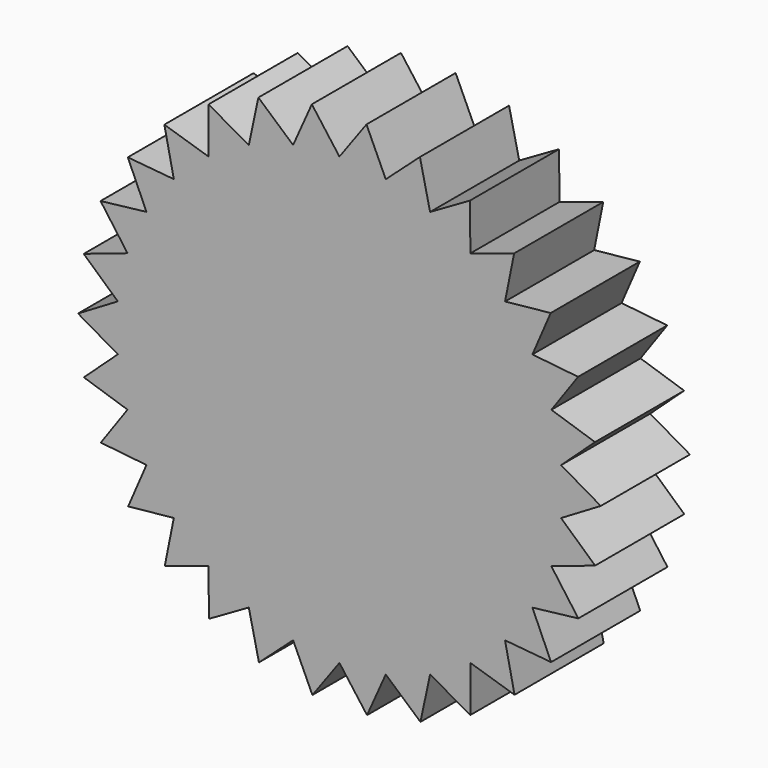
from build123d import *

# Parameters (mm, degrees)
F0_R            = 50.8
F1_DEPTH        = 12.7
F3_DEPTH        = 25.4
F3_COPIES_COUNT = 30


# Not quite as in the source:
# - a pattern or mirror of a feature is missing from the dataset's text; its kind, count and spacing are read off the source's solid


with BuildPart() as f1:
    # F0 (on Front) → F1 (new body, symmetric)
    with BuildSketch(Plane.XZ):
        Circle(F0_R)
    extrude(amount=F1_DEPTH, both=True)

    # F2 (on face) → F3 (join)
    with BuildSketch(Plane.XZ.offset(12.7)):
        with BuildLine():
            ThreePointArc((0, 50.8), (5.310045934, 50.5217122847), (10.5619138935, 49.6898981173))
            Line((10.5619138935, 49.6898981173), (6.1639756896, 59.2651665211))
            Line((6.1639756896, 59.2651665211), (0, 50.8))
        make_face()
    f3 = extrude(amount=-F3_DEPTH)

    # F3_copies: F3 ×30 about axis
    f3_copies_axis = Axis((0, 0, 0), (0, 1, 0))
    for i in range(1, F3_COPIES_COUNT):
        add(f3.rotate(f3_copies_axis, i * 360 / F3_COPIES_COUNT))


solid = f1.part
